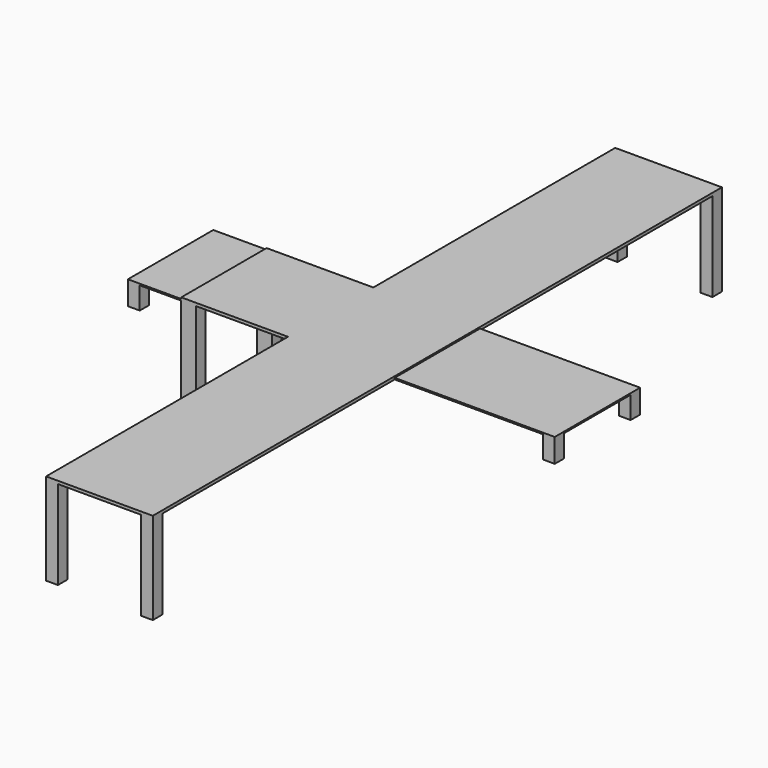
from build123d import *

# Parameters (mm, degrees)
F0_W     = 3657.6
F0_H     = 914.4
F1_DEPTH = 12.7
F2_W     = 101.6
F2_H     = 101.6
F3_DEPTH = 190.5
F4_W     = 914.4
F4_H     = 914.4
F5_DEPTH = 25
F6_W     = 101.6
F6_H     = 101.6
F6_W_2   = 125.4026571274
F7_DEPTH = 762


with BuildPart() as f1:
    # F0 (on Top) → F1 (new body)
    with BuildSketch(Plane.XY):
        Rectangle(F0_W, F0_H)
    extrude(amount=F1_DEPTH)

    # F2 (on face) → F3 (join)
    with BuildSketch(Plane(origin=(0, 0, 0), x_dir=(1, 0, 0), z_dir=(0, 0, -1))):
        with Locations((-1778, 406.4)):
            Rectangle(F2_W, F2_H)
        with Locations((1778, 406.4)):
            Rectangle(F2_W, F2_H)
        with Locations((-1778, -406.4)):
            Rectangle(F2_W, F2_H)
        with Locations((1778, -406.4)):
            Rectangle(F2_W, F2_H)
    extrude(amount=F3_DEPTH)


with BuildPart() as f5:
    # F4 (on Top) → F5 (new body)
    with BuildSketch(Plane.XY):
        Polygon((-457.2, -3048), (457.2, -3048), (457.2, 3048), (-457.2, 3048), (-457.2, 457.2), (-457.2, -457.2), align=None)
        with Locations((-914.4, 0)):
            Rectangle(F4_W, F4_H)
    extrude(amount=F5_DEPTH)

    # F6 (on face) → F7 (join)
    with BuildSketch(Plane(origin=(0, 0, 0), x_dir=(1, 0, 0), z_dir=(0, 0, -1))):
        with Locations((-406.4, 2997.2)):
            Rectangle(F6_W, F6_H)
        with Locations((406.4, 2997.2)):
            Rectangle(F6_W, F6_H)
        with Locations((-406.4, -2997.2)):
            Rectangle(F6_W, F6_H)
        with Locations((406.4, -2997.2)):
            Rectangle(F6_W, F6_H)
        with Locations((-1308.8986714363, 406.4)):
            Rectangle(F6_W_2, F6_H)
        with Locations((-1308.8986714363, -406.4)):
            Rectangle(F6_W_2, F6_H)
    extrude(amount=F7_DEPTH)


solid = Compound([f1.part, f5.part])
